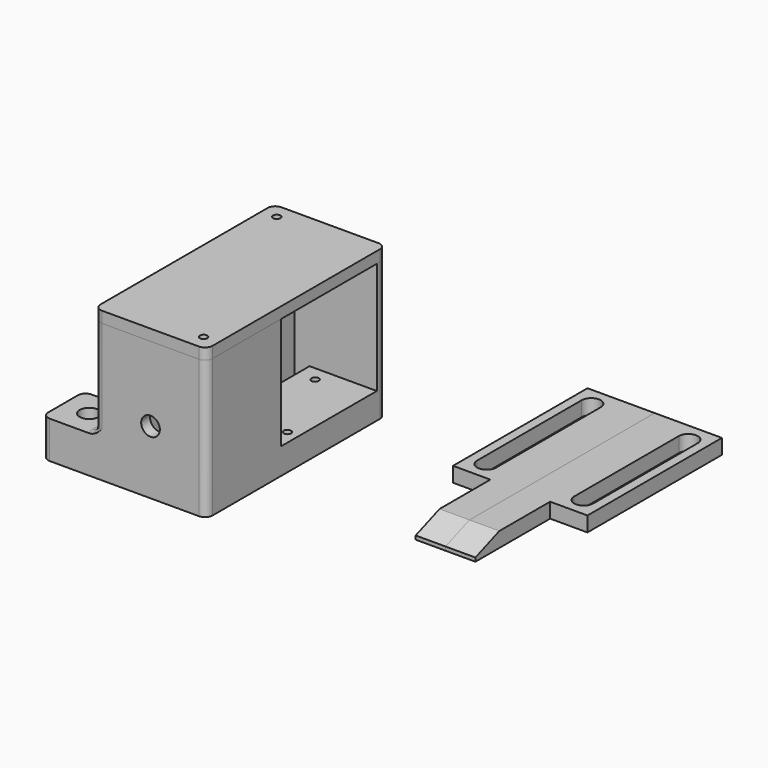
from build123d import *

# Parameters (mm, degrees)
F0_W          = 30
F0_H          = 60
F1_DEPTH      = 2
F3_DEPTH      = 35
F4_DEPTH      = 5
F6_D          = 2
F6_DEPTH      = 5
F6_TIP        = 0.600860619
F7_R          = 2
F8_W          = 5
F8_H          = 5
F9_DEPTH      = 35
F11_D         = 2
F11_DEPTH     = 14
F11_TIP       = 0.600860619
F12_R         = 2.5
F13_DEPTH     = 3
F15_DEPTH     = 10
F17_D         = 5.1054
F18_T1_DEPTH  = 10
F18_T3_DEPTH  = 12
F18_T5_DEPTH  = 12
F18_T10_ANGLE = 233.2969892374
F18_T15_ANGLE = 233.2969892374
F18_T22_DEPTH = 17
F18_T26_DEPTH = 15
F18_T33_DEPTH = 15
F18_T37_DEPTH = 17
F18_T40_DEPTH = 20
F19_R         = 1
F20_DEPTH     = 3
F22_DEPTH     = 4
F23_SIZE2     = 3
F23_SIZE      = 8


# Not quite as in the source:
# - a fillet or chamfer that OpenCascade refuses, or shapes differently, is made with other operations: its cross-section is extruded or revolved along the edge and cut away or added


with BuildPart() as f1:
    # F0 (on Top) → F1 (new body)
    with BuildSketch(Plane.XY):
        with Locations((15, 30)):
            Rectangle(F0_W, F0_H)
    extrude(amount=F1_DEPTH)

    # F2 (on face) → F3 (join)
    with BuildSketch(Plane.XY.offset(2)):
        Polygon((30, 60), (0, 60), (0, 0), (30, 0), (30, 25), (27, 25), (27, 3), (3, 3), (3, 57), (12, 57), (30, 57), align=None)
    extrude(amount=F3_DEPTH)

    # F2 (on face) → F4 (join)
    with BuildSketch(Plane.XY.offset(2)):
        Polygon((30, 25), (30, 57), (12, 57), (12, 25), (27, 25), align=None)
    extrude(amount=F4_DEPTH)

    # F6
    with Locations(Plane.XY.offset(7)):
        with Locations((16.7, 53), (27, 30.8)):
            Hole(F6_D / 2, depth=F6_DEPTH)
            with Locations((0, 0, -(F6_DEPTH + F6_TIP / 2))):  # 118° drill point
                Cone(0, F6_D / 2, F6_TIP, mode=Mode.SUBTRACT)

    # F7
    f7_edges = [f1.edges().sort_by_distance(p)[0] for p in [
        (30, 0, 18.5),
        (0, 0, 18.5),
        (0, 60, 18.5),
        (30, 60, 18.5),
    ]]
    fillet(f7_edges, radius=F7_R)

    # F8 (on face) → F9 (join, through all)
    with BuildSketch(Plane.XY.offset(2)):
        with Locations((5.5, 54.5)):
            Rectangle(F8_W, F8_H)
        with Locations((24.5, 5.5)):
            Rectangle(F8_W, F8_H)
    extrude(amount=F9_DEPTH)

    # F11
    with Locations(Plane.XY.offset(37)):
        with Locations((4, 56), (26, 4)):
            Hole(F11_D / 2, depth=F11_DEPTH)
            with Locations((0, 0, -(F11_DEPTH + F11_TIP / 2))):  # 118° drill point
                Cone(0, F11_D / 2, F11_TIP, mode=Mode.SUBTRACT)

    # F12 (on face) → F13 (cut, through all)
    with BuildSketch(Plane.XZ):
        with Locations((15, 17)):
            Circle(F12_R)
    extrude(amount=-F13_DEPTH, mode=Mode.SUBTRACT)

    # F14 (on face) → F15 (join)
    with BuildSketch(Plane(origin=(0, 0, 0), x_dir=(1, 0, 0), z_dir=(0, 0, -1))):
        with BuildLine():
            Line((0, -58), (0, -46))
            Line((0, -46), (-14, -46))
            Line((-14, -46), (-14, -60))
            Line((-14, -60), (2, -60))
            ThreePointArc((2, -60), (0.5857864376, -59.4142135624), (0, -58))
        make_face()
        with BuildLine():
            ThreePointArc((0, -2), (0.5857864376, -0.5857864376), (2, 0))
            Line((2, 0), (-14, 0))
            Line((-14, 0), (-14, -14))
            Line((-14, -14), (0, -14))
            Line((0, -14), (0, -2))
        make_face()
    extrude(amount=-F15_DEPTH)

    # F17 (through all)
    with Locations(Plane.XY.offset(10)):
        with Locations((-7, 53), (-7, 7)):
            Hole(F17_D / 2)

    # F18: fillet of radius 2 on 8 edges, made by hand

    # F18_s2 → F18_t1 (join)
    with BuildSketch(Plane.XY):
        with BuildLine():
            ThreePointArc((0, 44), (-0.5857864376, 45.4142135624), (-2, 46))
            Line((-2, 46), (0, 46))
            Line((0, 46), (0, 44))
        make_face()
        with BuildLine():
            ThreePointArc((0, 16), (-0.5857864376, 14.5857864376), (-2, 14))
            Line((-2, 14), (0, 14))
            Line((0, 14), (0, 16))
        make_face()
    extrude(amount=F18_T1_DEPTH)

    # F18_s4 → F18_t3 (join)
    with BuildSketch(Plane.XZ.offset(-14)):
        with BuildLine():
            ThreePointArc((0, 12), (-0.5857864376, 10.5857864376), (-2, 10))
            Line((-2, 10), (0, 10))
            Line((0, 10), (0, 12))
        make_face()
    extrude(amount=F18_T3_DEPTH)

    # F18_s6 → F18_t5 (join)
    with BuildSketch(Plane.XZ.offset(-58)):
        with BuildLine():
            ThreePointArc((0, 12), (-0.5857864376, 10.5857864376), (-2, 10))
            Line((-2, 10), (0, 10))
            Line((0, 10), (0, 12))
        make_face()
    extrude(amount=F18_T5_DEPTH)


with BuildPart() as f18_tool8:
    # F18_s9 → F18_t10 (revolve)
    with BuildSketch(Plane(origin=(29.0778128683, 21.6763107294, 0), x_dir=(0, 0, 1), z_dir=(-0.8017442393, -0.5976672776, 0))):
        with BuildLine():
            ThreePointArc((12, 43.305831324), (10.5857864376, 42.7200448864), (10, 41.305831324))
            Line((10, 41.305831324), (10, 43.305831324))
            Line((10, 43.305831324), (12, 43.305831324))
        make_face()
    revolve(axis=Axis((2, 58, 10), (0, 0, 1)), revolution_arc=F18_T10_ANGLE)

    split(bisect_by=Plane.XZ.offset(-60), keep=Keep.TOP)


with BuildPart() as f1_1:
    add(f1.part)

    # F18_t7: union F18_tool8
    add(f18_tool8.part)


with BuildPart() as f18_tool13:
    # F18_s14 → F18_t15 (revolve)
    with BuildSketch(Plane.XZ.offset(-2)):
        with BuildLine():
            ThreePointArc((-2, 10), (-0.5857864376, 10.5857864376), (0, 12))
            Line((0, 12), (0, 10))
            Line((0, 10), (-2, 10))
        make_face()
    revolve(axis=Axis((2, 2, 10), (0, 0, 1)), revolution_arc=F18_T15_ANGLE)

    split(bisect_by=Plane.XZ, keep=Keep.BOTTOM)

    split(bisect_by=Plane.XZ.offset(-3), keep=Keep.TOP)


with BuildPart() as f1_2:
    add(f1_1.part)

    # F18_t12: union F18_tool13
    add(f18_tool13.part)


with BuildPart() as f18_tool20:
    # F18_s21 → F18_t22 (new body)
    with BuildSketch(Plane.XZ.offset(-58)):
        with BuildLine():
            ThreePointArc((0, 12), (-0.5857864376, 10.5857864376), (-2, 10))
            Line((-2, 10), (0, 10))
            Line((0, 10), (0, 12))
        make_face()
    extrude(amount=F18_T22_DEPTH)

    split(bisect_by=Plane.XZ.offset(-46), keep=Keep.TOP)


with BuildPart() as f18_tool24:
    # F18_s25 → F18_t26 (new body)
    with BuildSketch(Plane.XY):
        with BuildLine():
            ThreePointArc((0, 44), (-0.5857864376, 45.4142135624), (-2, 46))
            Line((-2, 46), (0, 46))
            Line((0, 46), (0, 44))
        make_face()
    extrude(amount=F18_T26_DEPTH)

    split(bisect_by=Plane.XY.offset(10), keep=Keep.TOP)


with BuildPart() as f18_tool20_1:
    add(f18_tool20.part)

    # F18_t28: intersect F18_tool24
    add(f18_tool24.part, mode=Mode.INTERSECT)


with BuildPart() as f1_3:
    add(f1_2.part)

    # F18_t18: union F18_tool20
    add(f18_tool20_1.part)


with BuildPart() as f18_tool31:
    # F18_s32 → F18_t33 (new body)
    with BuildSketch(Plane.XY):
        with BuildLine():
            ThreePointArc((0, 16), (-0.5857864376, 14.5857864376), (-2, 14))
            Line((-2, 14), (0, 14))
            Line((0, 14), (0, 16))
        make_face()
    extrude(amount=F18_T33_DEPTH)

    split(bisect_by=Plane.XY.offset(10), keep=Keep.TOP)


with BuildPart() as f18_tool35:
    # F18_s36 → F18_t37 (new body)
    with BuildSketch(Plane.XZ.offset(-19)):
        with BuildLine():
            ThreePointArc((0, 12), (-0.5857864376, 10.5857864376), (-2, 10))
            Line((-2, 10), (0, 10))
            Line((0, 10), (0, 12))
        make_face()
    extrude(amount=F18_T37_DEPTH)

    split(bisect_by=Plane.XZ.offset(-14), keep=Keep.BOTTOM)


with BuildPart() as f18_tool31_1:
    add(f18_tool31.part)

    # F18_t39: intersect F18_tool35
    add(f18_tool35.part, mode=Mode.INTERSECT)


with BuildPart() as f1_4:
    add(f1_3.part)

    # F18_t29: union F18_tool31
    add(f18_tool31_1.part)

    # F18_s41 → F18_t40 (cut)
    with BuildSketch(Plane.XY.offset(-5)):
        with BuildLine():
            ThreePointArc((-14, 48), (-13.4142135624, 46.5857864376), (-12, 46))
            Line((-12, 46), (-14, 46))
            Line((-14, 46), (-14, 48))
        make_face()
        with BuildLine():
            ThreePointArc((-12, 60), (-13.4142135624, 59.4142135624), (-14, 58))
            Line((-14, 58), (-14, 60))
            Line((-14, 60), (-12, 60))
        make_face()
        with BuildLine():
            ThreePointArc((-12, 0), (-13.4142135624, 0.5857864376), (-14, 2))
            Line((-14, 2), (-14, 0))
            Line((-14, 0), (-12, 0))
        make_face()
        with BuildLine():
            ThreePointArc((-12, 14), (-13.4142135624, 13.4142135624), (-14, 12))
            Line((-14, 12), (-14, 14))
            Line((-14, 14), (-12, 14))
        make_face()
    extrude(amount=F18_T40_DEPTH, mode=Mode.SUBTRACT)


with BuildPart() as f20:
    # F19 (on face) → F20 (new body)
    with BuildSketch(Plane.XY.offset(37)):
        with BuildLine():
            Line((30, 2), (30, 25))
            Line((30, 25), (27, 25))
            Line((27, 25), (27, 8))
            Line((27, 8), (22, 8))
            Line((22, 8), (22, 3))
            Line((22, 3), (3, 3))
            Line((3, 3), (3, 52))
            Line((3, 52), (8, 52))
            Line((8, 52), (8, 57))
            Line((8, 57), (30, 57))
            Line((30, 57), (30, 58))
            ThreePointArc((30, 58), (29.4142135624, 59.4142135624), (28, 60))
            Line((28, 60), (2, 60))
            ThreePointArc((2, 60), (0.5857864376, 59.4142135624), (0, 58))
            Line((0, 58), (0, 2))
            ThreePointArc((0, 2), (0.5857864376, 0.5857864376), (2, 0))
            Line((2, 0), (28, 0))
            ThreePointArc((28, 0), (29.4142135624, 0.5857864376), (30, 2))
        make_face()
        with Locations((26, 4)):
            Circle(F19_R, mode=Mode.SUBTRACT)
        with Locations((4, 56)):
            Circle(F19_R, mode=Mode.SUBTRACT)
        Polygon((27, 25), (30, 25), (30, 57), (8, 57), (8, 52), (3, 52), (3, 3), (22, 3), (22, 8), (27, 8), align=None)
    extrude(amount=F20_DEPTH)


with BuildPart() as f22:
    # F21 (on Top) → F22 (new body)
    with BuildSketch(Plane.XY):
        Polygon((70, 45), (70, 20), (78, 20), (78, 90), (60, 90), (60, 45), align=None)
        with BuildLine():
            ThreePointArc((62.4473, 85), (65, 87.5527), (67.5527, 85))
            Line((67.5527, 85), (67.5527, 50))
            ThreePointArc((67.5527, 50), (65, 47.4473), (62.4473, 50))
            Line((62.4473, 50), (62.4473, 85))
        make_face(mode=Mode.SUBTRACT)
    extrude(amount=F22_DEPTH)

    # F23
    f23_edges = [f22.edges().sort_by_distance(p)[0] for p in [
        (74, 20, 4),
    ]]
    f23_side = f22.faces().sort_by_distance((71.21578, 58.866972, 4))[0]
    chamfer(f23_edges, length=F23_SIZE, length2=F23_SIZE2, reference=f23_side)


with BuildPart() as f24_1:
    # F24: instance of F22
    add(f22.part.mirror(Plane(origin=(78, 56.447761194, 1.9552238806), x_dir=(0, 1, 0), z_dir=(1, 0, 0))))


solid = Compound([f1_4.part, f20.part, f22.part, f24_1.part])
